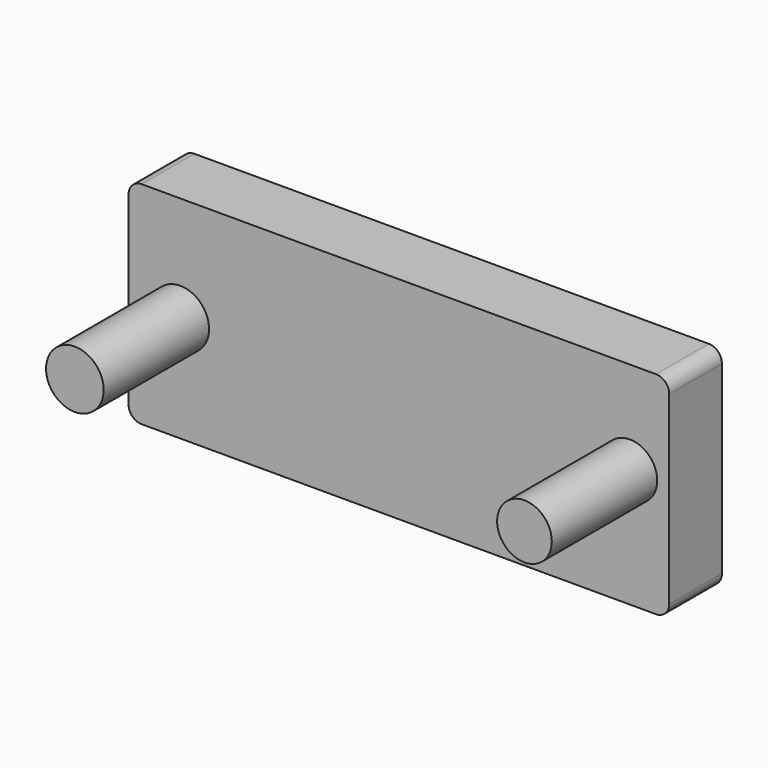
from build123d import *

# Parameters (mm, degrees)
F0_W     = 208.4420993924
F0_H     = 81.4700946212
F1_DEPTH = 25.4
F2_R     = 11.1076712279
F2_R_2   = 10.5439005504
F3_DEPTH = 50.8
F7_R     = 5.08


# Not quite as in the source:
# - the program builds the solid bodies; features that only make, move or delete a surface that nothing else refers to are left out


with BuildPart() as f1:
    # F0 (on Front) → F1 (new body)
    with BuildSketch(Plane.XZ):
        with Locations((-3.9001591504, -4.76687029)):
            Rectangle(F0_W, F0_H)
    extrude(amount=F1_DEPTH)

    # F2 (on face) → F3 (join)
    with BuildSketch(Plane.XZ.offset(25.4)):
        with Locations((-88.1870388985, -4.7668707557)):
            Circle(F2_R)
        with Locations((85.1535871625, 0)):
            Circle(F2_R_2)
    extrude(amount=F3_DEPTH)

    # F7
    f7_edges = [f1.edges().sort_by_distance(p)[0] for p in [
        (100.320891, -12.7, -45.501918),
        (-108.121209, -12.7, -45.501918),
        (-108.121209, -12.7, 35.968177),
        (100.320891, -12.7, 35.968177),
    ]]
    fillet(f7_edges, radius=F7_R)


solid = f1.part
